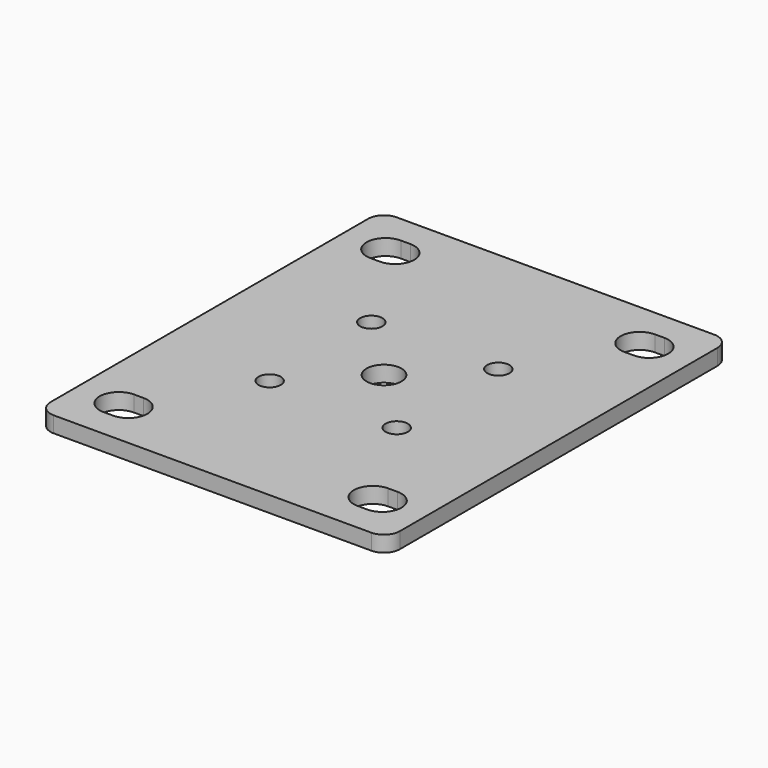
from build123d import *

# Parameters (mm, degrees)
F0_W             = 110
F0_H             = 135
F1_DEPTH         = 5
F2_R             = 3.5
F2_R_2           = 5.5
F3_DEPTH         = 25
F5_DEPTH         = 25
F5_COPIES2_COUNT = 2
F5_COPIES2_PITCH = 132.003788
F6_R             = 5


# Not quite as in the source:
# - a pattern or mirror of a feature is missing from the dataset's text; its kind, count and spacing are read off the source's solid


with BuildPart() as f1:
    # F0 (on Top) → F1 (new body)
    with BuildSketch(Plane.XY):
        Rectangle(F0_W, F0_H)
    extrude(amount=F1_DEPTH)

    # F2 (on face) → F3 (cut)
    with BuildSketch(Plane.XY.offset(5)):
        with Locations((-20, 20)):
            Circle(F2_R)
        with Locations((20, 20)):
            Circle(F2_R)
        with Locations((20, -20)):
            Circle(F2_R)
        with Locations((-20, -20)):
            Circle(F2_R)
        Circle(F2_R_2)
    extrude(amount=-F3_DEPTH, mode=Mode.SUBTRACT)

    # F4 (on face) → F5 (cut)
    with BuildSketch(Plane.XY.offset(5)):
        with BuildLine():
            ThreePointArc((-41.5, 58.5), (-47.5, 52.5), (-41.5, 46.5))
            Line((-41.5, 46.5), (-38.5, 46.5))
            ThreePointArc((-38.5, 46.5), (-32.5, 52.5), (-38.5, 58.5))
            Line((-38.5, 58.5), (-41.5, 58.5))
        make_face()
    f5 = extrude(amount=-F5_DEPTH, mode=Mode.SUBTRACT)

    # F5_copies: F5 across plane
    add(f5.mirror(Plane(origin=(0, 0, 0), x_dir=(0, 0, -1), z_dir=(0, -1, 0))), mode=Mode.SUBTRACT)

    # F5_copies1: F5 across plane
    add(f5.mirror(Plane(origin=(0, 0, 0), x_dir=(0, 0, 1), z_dir=(1, 0, 0))), mode=Mode.SUBTRACT)

    # F5_copies2: F5 ×2
    with Locations(*[Vector(0.6060432153, -0.79543172, 0) * (i * F5_COPIES2_PITCH) for i in range(1, F5_COPIES2_COUNT)]):
        add(f5, mode=Mode.SUBTRACT)

    # F6
    f6_edges = [f1.edges().sort_by_distance(p)[0] for p in [
        (-55, 67.5, 2.5),
        (55, 67.5, 2.5),
        (55, -67.5, 2.5),
        (-55, -67.5, 2.5),
    ]]
    fillet(f6_edges, radius=F6_R)


solid = f1.part
